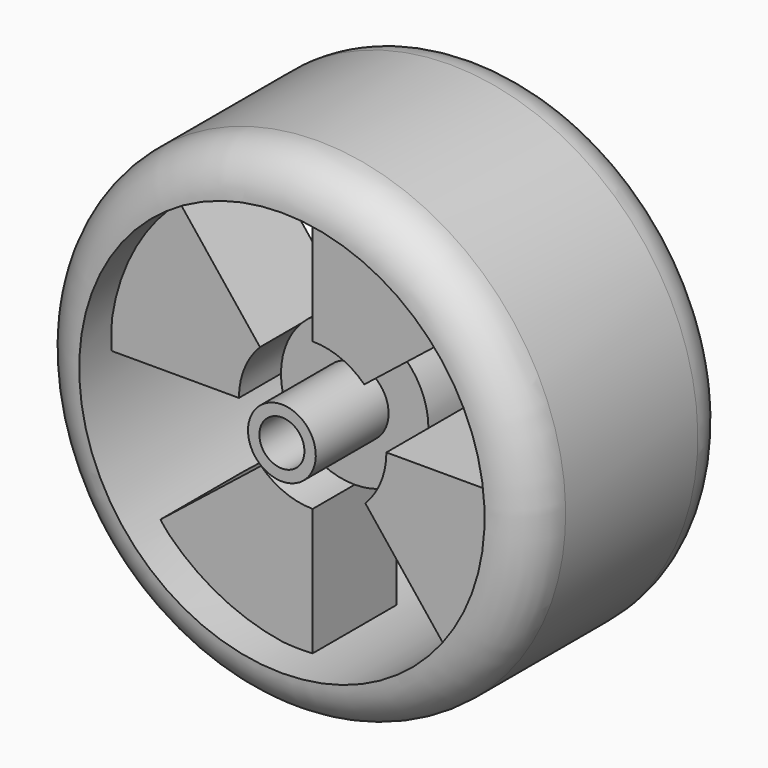
from build123d import *

# Parameters (mm, degrees)
F0_W     = 17
F0_H     = 3
F3_DEPTH = 3.5
F4_COUNT = 4
F5_R     = 2.99999


# Not quite as in the source:
# - a fillet or chamfer is up to 0.001 mm smaller than in the source, because OpenCascade refuses the exact size


with BuildPart() as f1:
    # F0 (on Right) → F1 (revolve)
    with BuildSketch(Plane.YZ):
        with Locations((8.5, 15)):
            Rectangle(F0_W, F0_H)
    revolve(axis=Axis((0, 4.8521989956, 0), (0, 1, 0)))



with BuildPart() as f1b:
    # F0 (on Right) → F1, piece 2 (revolve)
    with BuildSketch(Plane.YZ):
        Polygon((0, 2.2574728355), (0, 1.5), (9.8266890272, 1.5), (9.8266890272, 4.9105980434), (6.0609620996, 4.9105980434), (6.0609620996, 2.2574728355), align=None)
    revolve(axis=Axis((0, 4.8521989956, 0), (0, 1, 0)))


with BuildPart() as f1_1:
    add(f1.part)

    add(f1b.part)  # F3 merges F1b
    # F2 (on face) → F3 (join, symmetric)
    with BuildSketch(Plane.XZ.offset(-6.0609620996)):
        with BuildLine():
            Line((0, 13.3796269074), (0, 4.9105980434))
            ThreePointArc((0, 4.9105980434), (1.8559366755, 4.5463691227), (3.4365562486, 3.5077135421))
            Line((3.4365562486, 3.5077135421), (10.1425750181, 8.8311284781))
            ThreePointArc((10.1425750181, 8.8311284781), (5.6432817311, 12.3808523131), (0, 13.3796269074))
        make_face()
    extrude(amount=F3_DEPTH, both=True)

    # F4: F1 ×4 about axis
    f4_axis = Axis((0, 9.8266890272, 0), (0, 1, 0))


with BuildPart() as f1_2:
    add(f1_1.part)
    for i in range(1, F4_COUNT):
        add(f1_1.part.rotate(f4_axis, i * 360 / F4_COUNT))

    # F5 (radius 3 in the source; OpenCascade refuses exactly that, so slightly less here)
    f5_edges = [f1_2.edges().sort_by_distance(p)[0] for p in [
        (0, 0, -16.5),
        (0, 17, -16.5),
    ]]
    fillet(f5_edges, radius=F5_R)


solid = f1_2.part
